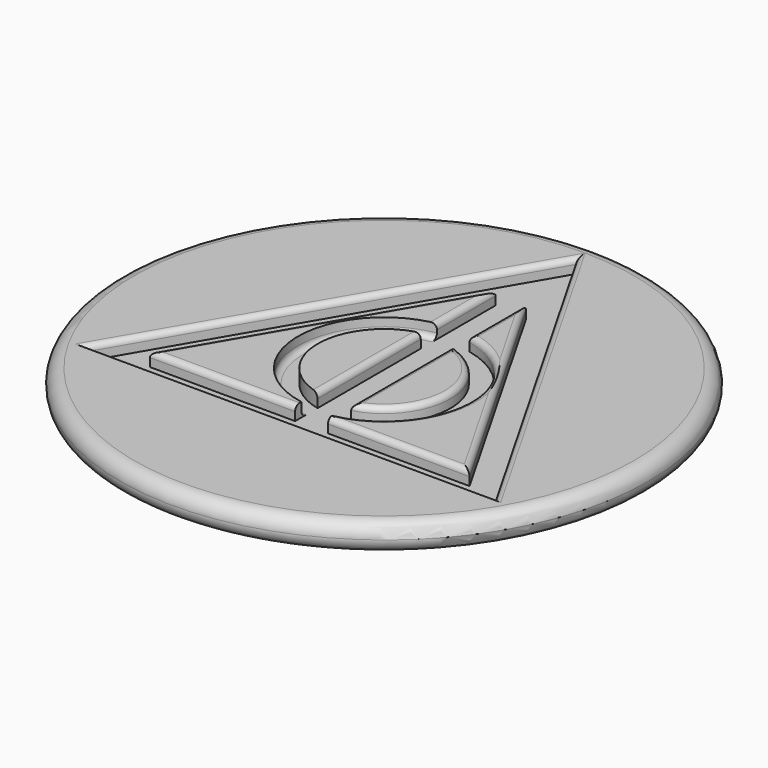
from build123d import *

# Parameters (mm, degrees)
F0_R         = 47.5
F1_DEPTH     = 5
F3_DEPTH     = 2.5
F4_R         = 15.4938561144
F4_R_2       = 11.9238234347
F5_DEPTH     = 2.5
F7_DEPTH     = 2.5
F8_R         = 2.49999
F9_T1_DEPTH  = 79.5044599257
F9_T6_ANGLE  = 178.5086872517
F9_T8_DEPTH  = 27.9406148573
F9_T10_DEPTH = 28.2323532374
F9_T12_DEPTH = 17.7111990238
F9_T14_DEPTH = 18.2220956401
F9_T16_DEPTH = 31.2335819135
F9_T18_DEPTH = 30.5369030224
F9_T20_DEPTH = 56.4226854656
F9_T22_DEPTH = 57.113596888
F9_T25_ANGLE = 172.3459061433
F9_T27_ANGLE = 174.2406786555
F9_T31_DEPTH = 79.5044599257
F9_T37_DEPTH = 79.5044599257
F9_T44_DEPTH = 79.5044599257
F9_T48_DEPTH = 79.5044599257


# Not quite as in the source:
# - a fillet or chamfer that OpenCascade refuses, or shapes differently, is made with other operations: its cross-section is extruded or revolved along the edge and cut away or added
# - a fillet or chamfer is up to 0.001 mm smaller than in the source, because OpenCascade refuses the exact size


with BuildPart() as f1:
    # F0 (on Top) → F1 (new body)
    with BuildSketch(Plane.XY):
        Circle(F0_R)
    extrude(amount=F1_DEPTH)

    # F2 (on face) → F3 (cut)
    with BuildSketch(Plane.XY.offset(5)):
        Polygon((-37.336189985, -21.3615019839), (37.1676983736, -21.6533380156), (0.1684916114, 43.0148399995), align=None)
        Polygon((-28.924478218, -16.5488310158), (0.1305310463, 33.3237484359), (28.7939471716, -16.77491742), align=None, mode=Mode.SUBTRACT)
    extrude(amount=-F3_DEPTH, mode=Mode.SUBTRACT)

    # F4 (on face) → F5 (cut)
    with BuildSketch(Plane.XY.offset(5)):
        Circle(F4_R)
        Circle(F4_R_2, mode=Mode.SUBTRACT)
    extrude(amount=-F5_DEPTH, mode=Mode.SUBTRACT)

    # F6 (on face) → F7 (cut)
    with BuildSketch(Plane.XY.offset(5)):
        with BuildLine():
            Line((3.2572400577, 27.8588049238), (0.1305310463, 33.3237484359))
            Line((0.1305310463, 33.3237484359), (-2.6910975575, 28.4804563395))
            Line((-2.6910975575, 28.4804563395), (-2.6910975575, 15.2583606993))
            ThreePointArc((-2.6910975575, 15.2583606993), (0.2884371491, 15.491171076), (3.2572400577, 15.1476059))
            Line((3.2572400577, 15.1476059), (3.2572400577, 27.8588049238))
        make_face()
        with BuildLine():
            ThreePointArc((3.2572400577, 15.1476059), (0.2884371491, 15.491171076), (-2.6910975575, 15.2583606993))
            Line((-2.6910975575, 15.2583606993), (-2.6910975575, -15.2583606993))
            ThreePointArc((-2.6910975575, -15.2583606993), (0.2884371491, -15.491171076), (3.2572400577, -15.1476059))
            Line((3.2572400577, -15.1476059), (3.2572400577, 15.1476059))
        make_face()
        with BuildLine():
            ThreePointArc((3.2572400577, -15.1476059), (0.2884371491, -15.491171076), (-2.6910975575, -15.2583606993))
            Line((-2.6910975575, -15.2583606993), (-2.6910975575, -16.6515886823))
            Line((-2.6910975575, -16.6515886823), (3.2572400577, -16.6748886641))
            Line((3.2572400577, -16.6748886641), (3.2572400577, -15.1476059))
        make_face()
    extrude(amount=-F7_DEPTH, mode=Mode.SUBTRACT)

    # F8 (radius 2.5 in the source; OpenCascade refuses exactly that, so slightly less here)
    f8_edges = [f1.edges().sort_by_distance(p)[0] for p in [
        (-47.5, 0, 5),
        (-47.5, 0, 0),
    ]]
    fillet(f8_edges, radius=F8_R)

    # F9: fillet of radius 1 on 14 edges, made by hand

    # F9_s2 → F9_t1 (join)
    with BuildSketch(Plane(origin=(-39.7519250003, 0.155710585, 0), x_dir=(0, 0, 1), z_dir=(0.9999923284, -0.0039170277, 0))):
        with BuildLine():
            ThreePointArc((3.5, 21.507584997), (2.7928932188, 21.2146917781), (2.5, 20.507584997))
            Line((2.5, 20.507584997), (2.5, 21.507584997))
            Line((2.5, 21.507584997), (3.5, 21.507584997))
        make_face()
    extrude(amount=F9_T1_DEPTH)


with BuildPart() as f9_tool4:
    # F9_s5 → F9_t6 (revolve)
    with BuildSketch(Plane(origin=(0, 0, 0), x_dir=(0, 0, 1), z_dir=(0.999915317, 0.0130137915, 0))):
        with BuildLine():
            ThreePointArc((2.5, -14.4938561144), (2.7928932188, -15.2009628956), (3.5, -15.4938561144))
            Line((3.5, -15.4938561144), (2.5, -15.4938561144))
            Line((2.5, -15.4938561144), (2.5, -14.4938561144))
        make_face()
    revolve(axis=Axis((0, 0, 2.5), (0, 0, 1)), revolution_arc=F9_T6_ANGLE)

    split(bisect_by=Plane.YZ.offset(-2.6910975575), keep=Keep.BOTTOM)


with BuildPart() as f1_1:
    add(f1.part)

    # F9_t3: union F9_tool4
    add(f9_tool4.part)

    # F9_s9 → F9_t8 (cut)
    with BuildSketch(Plane.XZ.offset(-13.9703074287)):
        with BuildLine():
            ThreePointArc((4.2572400577, 5), (3.5501332765, 4.7071067812), (3.2572400577, 4))
            Line((3.2572400577, 4), (3.2572400577, 5))
            Line((3.2572400577, 5), (4.2572400577, 5))
        make_face()
    extrude(amount=F9_T8_DEPTH, mode=Mode.SUBTRACT)

    # F9_s11 → F9_t10 (cut)
    with BuildSketch(Plane.XZ.offset(-14.1161766187)):
        with BuildLine():
            ThreePointArc((-2.6910975575, 4), (-2.9839907764, 4.7071067812), (-3.6910975575, 5))
            Line((-3.6910975575, 5), (-2.6910975575, 5))
            Line((-2.6910975575, 5), (-2.6910975575, 4))
        make_face()
    extrude(amount=F9_T10_DEPTH, mode=Mode.SUBTRACT)

    # F9_s13 → F9_t12 (cut)
    with BuildSketch(Plane.XZ.offset(-30.3588049238)):
        with BuildLine():
            ThreePointArc((4.2572400577, 5), (3.5501332765, 4.7071067812), (3.2572400577, 4))
            Line((3.2572400577, 4), (3.2572400577, 5))
            Line((3.2572400577, 5), (4.2572400577, 5))
        make_face()
    extrude(amount=F9_T12_DEPTH, mode=Mode.SUBTRACT)

    # F9_s15 → F9_t14 (cut)
    with BuildSketch(Plane.XZ.offset(-30.9804563395)):
        with BuildLine():
            ThreePointArc((-3.6910975575, 5), (-2.9839907764, 4.7071067812), (-2.6910975575, 4))
            Line((-2.6910975575, 4), (-2.6910975575, 5))
            Line((-2.6910975575, 5), (-3.6910975575, 5))
        make_face()
    extrude(amount=F9_T14_DEPTH, mode=Mode.SUBTRACT)

    # F9_s17 → F9_t16 (cut)
    with BuildSketch(Plane(origin=(-0.1258512133, 0.0004929665, 0), x_dir=(0, 0, 1), z_dir=(-0.9999923284, 0.0039170277, 0))):
        with BuildLine():
            ThreePointArc((5, -15.6620020419), (4.7071067812, -16.369108823), (4, -16.6620020419))
            Line((4, -16.6620020419), (5, -16.6620020419))
            Line((5, -16.6620020419), (5, -15.6620020419))
        make_face()
    extrude(amount=F9_T16_DEPTH, mode=Mode.SUBTRACT)

    # F9_s19 → F9_t18 (cut)
    with BuildSketch(Plane(origin=(31.3591935158, -0.1228357713, 0), x_dir=(0, 0, 1), z_dir=(-0.9999923284, 0.0039170277, 0))):
        with BuildLine():
            ThreePointArc((5, -15.6620020419), (4.7071067812, -16.369108823), (4, -16.6620020419))
            Line((4, -16.6620020419), (5, -16.6620020419))
            Line((5, -16.6620020419), (5, -15.6620020419))
        make_face()
    extrude(amount=F9_T18_DEPTH, mode=Mode.SUBTRACT)

    # F9_s21 → F9_t20 (cut)
    with BuildSketch(Plane(origin=(-12.4465088481, 21.7543326005, 0), x_dir=(0, 0, 1), z_dir=(0.4966039187, -0.8679772738, 0))):
        with BuildLine():
            ThreePointArc((4, -16.6620020419), (4.7071067812, -16.369108823), (5, -15.6620020419))
            Line((5, -15.6620020419), (5, -16.6620020419))
            Line((5, -16.6620020419), (4, -16.6620020419))
        make_face()
    extrude(amount=F9_T20_DEPTH, mode=Mode.SUBTRACT)

    # F9_s23 → F9_t22 (cut)
    with BuildSketch(Plane(origin=(-15.7859756564, -27.0964403413, 0), x_dir=(0, 0, 1), z_dir=(0.5033884097, 0.8640602462, 0))):
        with BuildLine():
            ThreePointArc((5, -15.6620020419), (4.7071067812, -16.369108823), (4, -16.6620020419))
            Line((4, -16.6620020419), (5, -16.6620020419))
            Line((5, -16.6620020419), (5, -15.6620020419))
        make_face()
    extrude(amount=F9_T22_DEPTH, mode=Mode.SUBTRACT)

    # F9_s24 → F9_t25 (revolve, cut)
    with BuildSketch(Plane(origin=(0, 0, 0), x_dir=(0, 0, 1), z_dir=(-0.997770072, 0.0667449131, 0))):
        with BuildLine():
            ThreePointArc((4, 11.9238234347), (4.7071067812, 11.6309302159), (5, 10.9238234347))
            Line((5, 10.9238234347), (5, 11.9238234347))
            Line((5, 11.9238234347), (4, 11.9238234347))
        make_face()
    revolve(axis=Axis((0, 0, 5), (0, 0, -1)), revolution_arc=F9_T25_ANGLE, mode=Mode.SUBTRACT)

    # F9_s26 → F9_t27 (revolve, cut)
    with BuildSketch(Plane(origin=(0, 0, 0), x_dir=(0, 0, 1), z_dir=(-0.9987372542, 0.0502384033, 0))):
        with BuildLine():
            ThreePointArc((5, 16.4938561144), (4.7071067812, 15.7867493333), (4, 15.4938561144))
            Line((4, 15.4938561144), (5, 15.4938561144))
            Line((5, 15.4938561144), (5, 16.4938561144))
        make_face()
    revolve(axis=Axis((0, 0, 5), (0, 0, -1)), revolution_arc=F9_T27_ANGLE, mode=Mode.SUBTRACT)


with BuildPart() as f9_tool29:
    # F9_s30 → F9_t31 (new body)
    with BuildSketch(Plane(origin=(20.0108118224, 34.3483216071, 0), x_dir=(0, 0, 1), z_dir=(-0.5033884097, -0.8640602462, 0))):
        with BuildLine():
            ThreePointArc((5, 22.507584997), (4.7071067812, 21.8004782158), (4, 21.507584997))
            Line((4, 21.507584997), (5, 21.507584997))
            Line((5, 21.507584997), (5, 22.507584997))
        make_face()
    extrude(amount=F9_T31_DEPTH)

    split(bisect_by=Plane(origin=(18.6680949925, 10.680750992, 0), x_dir=(0, 0, 1), z_dir=(-0.8679772738, -0.4966039187, 0)), keep=Keep.TOP)

    split(bisect_by=Plane(origin=(-0.0842458057, -21.5074199997, 0), x_dir=(0, 0, 1), z_dir=(0.0039170277, 0.9999923284, 0)), keep=Keep.TOP)


with BuildPart() as f1_2:
    add(f1_1.part)

    # F9_t28: cut F9_tool29
    add(f9_tool29.part, mode=Mode.SUBTRACT)


with BuildPart() as f9_tool35:
    # F9_s36 → F9_t37 (new body)
    with BuildSketch(Plane(origin=(19.7411131779, -34.5040321921, 0), x_dir=(0, 0, 1), z_dir=(-0.4966039187, 0.8679772738, 0))):
        with BuildLine():
            ThreePointArc((5, 22.507584997), (4.7071067812, 21.8004782158), (4, 21.507584997))
            Line((4, 21.507584997), (5, 21.507584997))
            Line((5, 21.507584997), (5, 22.507584997))
        make_face()
    extrude(amount=F9_T37_DEPTH)

    split(bisect_by=Plane(origin=(-18.5838491868, 10.8266690078, 0), x_dir=(0, 0, 1), z_dir=(0.8640602462, -0.5033884097, 0)), keep=Keep.TOP)

    split(bisect_by=Plane(origin=(-0.0842458057, -21.5074199997, 0), x_dir=(0, 0, 1), z_dir=(0.0039170277, 0.9999923284, 0)), keep=Keep.TOP)


with BuildPart() as f1_3:
    add(f1_2.part)

    # F9_t34: cut F9_tool35
    add(f9_tool35.part, mode=Mode.SUBTRACT)


with BuildPart() as f9_tool42:
    # F9_s43 → F9_t44 (new body)
    with BuildSketch(Plane(origin=(20.0108118224, 34.3483216071, 0), x_dir=(0, 0, 1), z_dir=(-0.5033884097, -0.8640602462, 0))):
        with BuildLine():
            ThreePointArc((5, 22.507584997), (4.7071067812, 21.8004782158), (4, 21.507584997))
            Line((4, 21.507584997), (5, 21.507584997))
            Line((5, 21.507584997), (5, 22.507584997))
        make_face()
    extrude(amount=F9_T44_DEPTH)

    split(bisect_by=Plane(origin=(18.6680949925, 10.680750992, 0), x_dir=(0, 0, 1), z_dir=(0.8679772738, 0.4966039187, 0)), keep=Keep.TOP)


with BuildPart() as f9_tool46:
    # F9_s47 → F9_t48 (new body)
    with BuildSketch(Plane(origin=(19.7411131779, -34.5040321921, 0), x_dir=(0, 0, 1), z_dir=(-0.4966039187, 0.8679772738, 0))):
        with BuildLine():
            ThreePointArc((5, 22.507584997), (4.7071067812, 21.8004782158), (4, 21.507584997))
            Line((4, 21.507584997), (5, 21.507584997))
            Line((5, 21.507584997), (5, 22.507584997))
        make_face()
    extrude(amount=F9_T48_DEPTH)

    split(bisect_by=Plane(origin=(-18.5838491868, 10.8266690078, 0), x_dir=(0, 0, 1), z_dir=(-0.8640602462, 0.5033884097, 0)), keep=Keep.TOP)


with BuildPart() as f9_tool42_1:
    add(f9_tool42.part)

    # F9_t50: intersect F9_tool46
    add(f9_tool46.part, mode=Mode.INTERSECT)


with BuildPart() as f1_4:
    add(f1_3.part)

    # F9_t40: cut F9_tool42
    add(f9_tool42_1.part, mode=Mode.SUBTRACT)


solid = f1_4.part
